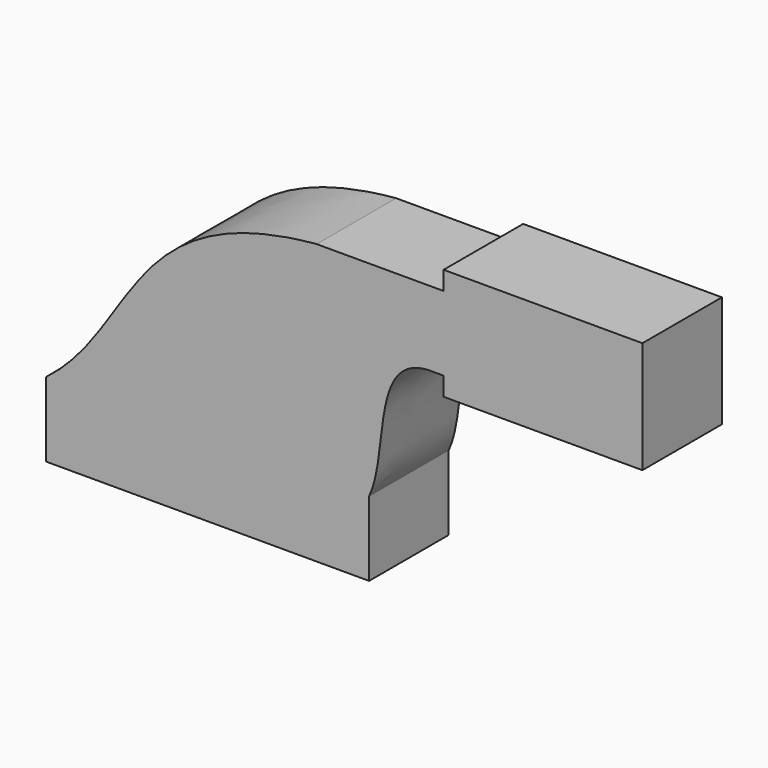
from build123d import *

# Parameters (mm, degrees)
F0_W     = 23.8088733172
F0_H     = 19.05
F1_DEPTH = 25.4


# Not quite as in the source:
# - ends of sketch curves that miss each other by under 0.0002 mm in the source are joined


with BuildPart() as f1:
    # F0 (on Front) → F1 (new body)
    with BuildSketch(Plane.XZ):
        Polygon((-41.275, -9.525), (41.275, -9.525), (41.275, 9.525), (22.225, 9.525), (-41.275, 9.525), align=None)
        with BuildLine():
            Line((22.225, 9.525), (41.275, 9.525))
            Line((41.275, 9.525), (41.275, 42.8498))
            Line((41.275, 42.8498), (56.2650781978, 42.8498))
            Line((56.2650781978, 42.8498), (60.325, 42.8498))
            Line((60.325, 42.8498), (60.325, 61.8998))
            Line((60.325, 61.8998), (27.8614319257, 61.8998))
            ThreePointArc((27.8614319257, 61.8998), (23.6637426323, 52.7961975559), (22.225, 42.8752))
            Line((22.225, 42.8752), (22.225, 9.525))
        make_face()
        with BuildLine():
            Line((41.275, 42.8498), (41.275, 9.525))
            add(Edge.make_bspline(
                [(56.2650781978, 42.8498), (41.47290193, 42.0072197884), (46.465802928, 20.4298387912), (41.275, 9.525)],
                knots=[0.7040277811, 0.7040277811, 0.7040277811, 0.7040277811, 36.9357748672, 36.9357748672, 36.9357748672, 36.9357748672], degree=3))
            Line((56.2650781978, 42.8498), (41.275, 42.8498))
        make_face()
        with BuildLine():
            add(Edge.make_bspline(
                [(-41.275, 9.525), (-18.2295226914, 26.9832666667), (-20.9687221795, 57.534776628), (27.8614319257, 61.8998)],
                knots=[0, 0, 0, 0, 86.7350326827, 86.7350326827, 86.7350326827, 86.7350326827], degree=3))
            Line((-41.275, 9.525), (22.225, 9.525))
            Line((22.225, 9.525), (22.225, 42.8752))
            ThreePointArc((22.225, 42.8752), (23.6637426323, 52.7961975559), (27.8614319257, 61.8998))
        make_face()
        Polygon((84.1338733172, 42.8498), (60.325, 42.8498), (60.325, 38.1), (111.125, 38.1), (111.125, 66.675), (60.325, 66.675), (60.325, 61.8998), (84.1338733172, 61.8998), align=None)
        with Locations((72.2294366586, 52.3748)):
            Rectangle(F0_W, F0_H)
    extrude(amount=F1_DEPTH)


solid = f1.part
